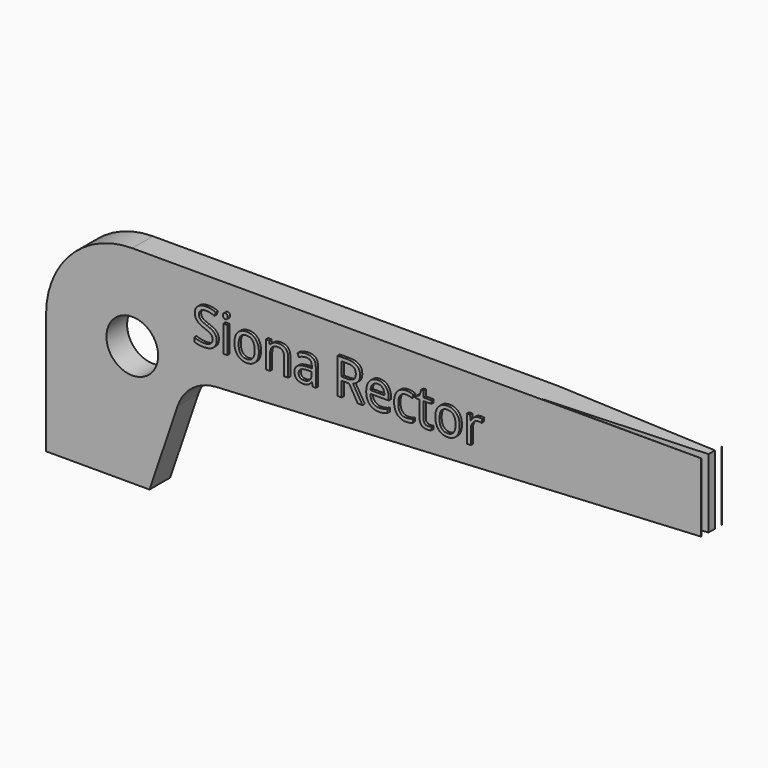
from build123d import *

# Parameters (mm, degrees)
F1_DEPTH     = 2.38125
F2_R         = 2.38125
F3_DEPTH     = 25.4
F6_DEPTH     = 25.4
F7_R         = 2.38125
F7_W         = 0.4099813808
F7_H         = 2.7055611352
F8_DEPTH     = 0.254
F9_TEXT_SIZE = 4.5757921827
F10_DEPTH    = 0.254


# Not quite as in the source:
# - Text() gives the source's letters only with a copy of the font that has no kerning and outlines rounded to 1/6400 em; it was checked with that copy


with BuildPart() as f1:
    # F0 (on Front) → F1 (new body)
    with BuildSketch(Plane.XZ):
        with BuildLine():
            Line((60.325, 19.05), (7.9375, 19.05))
            ThreePointArc((7.9375, 19.05), (2.3248399243, 16.7251600757), (0, 11.1125))
            Line((0, 11.1125), (0, 0))
            Line((0, 0), (9.525, 0))
            Line((9.525, 0), (12.1173647876, 7.6271664624))
            ThreePointArc((12.1173647876, 7.6271664624), (13.4786145605, 9.5135918491), (15.6631963617, 10.3130942181))
            Line((15.6631963617, 10.3130942181), (60.325, 12.7))
            Line((60.325, 12.7), (60.325, 19.05))
        make_face()
    extrude(amount=F1_DEPTH)

    # F2 (on face) → F3 (cut)
    with BuildSketch(Plane.XZ.offset(2.38125)):
        with Locations((7.9375, 11.1125)):
            Circle(F2_R)
    extrude(amount=-F3_DEPTH, mode=Mode.SUBTRACT)

    # F5 (on face) → F6 (cut)
    with BuildSketch(Plane.XY.offset(19.05)):
        Polygon((60.3245161474, 0), (45.24375, 0), (60.3431798518, -0.79375), align=None)
        Polygon((60.3431798518, -1.5423499767), (45.24375, -2.3360999767), (60.3328719735, -2.377419034), align=None)
    extrude(amount=-F6_DEPTH, mode=Mode.SUBTRACT)

    # F7 (on face) → F8 (cut)
    with BuildSketch(Plane.XZ.offset(2.38125)):
        with BuildLine():
            ThreePointArc((12.1173647876, 7.6271664624), (13.4786145605, 9.5135918491), (15.6631963617, 10.3130942181))
            Line((15.6631963617, 10.3130942181), (60.325, 12.7))
            Line((60.325, 12.7), (60.325, 19.05))
            Line((60.325, 19.05), (7.9375, 19.05))
            ThreePointArc((7.9375, 19.05), (2.3248399243, 16.7251600757), (0, 11.1125))
            Line((0, 11.1125), (0, 0))
            Line((0, 0), (9.525, 0))
            Line((9.525, 0), (12.1173647876, 7.6271664624))
        make_face()
        with Locations((7.9375, 11.1125)):
            Circle(F7_R, mode=Mode.SUBTRACT)
        with Locations((17.9440042047, 14.4853611236)):
            Rectangle(F7_W, F7_H, mode=Mode.SUBTRACT)
        with BuildLine():
            add(Edge.make_bspline(
                [(16.8487456605, 14.6950914831), (17.0620307718, 14.4628476951), (17.0620307718, 14.0931535021)],
                knots=[0, 0, 0, 1, 1, 1], degree=2))
            add(Edge.make_bspline(
                [(17.0620307718, 14.0931535021), (17.0620307718, 13.6168167533), (16.7164298969, 13.3498153916)],
                knots=[0, 0, 0, 1, 1, 1], degree=2))
            add(Edge.make_bspline(
                [(16.7164298969, 13.3498153916), (16.370829022, 13.08281403), (15.7783703792, 13.08281403)],
                knots=[0, 0, 0, 1, 1, 1], degree=2))
            add(Edge.make_bspline(
                [(15.7783703792, 13.08281403), (15.1369351554, 13.08281403), (14.790939308, 13.24870245)],
                knots=[0, 0, 0, 1, 1, 1], degree=2))
            Line((14.790939308, 13.24870245), (14.790939308, 13.6531542167))
            add(Edge.make_bspline(
                [(14.790939308, 13.6531542167), (15.0137037577, 13.5599407236), (15.2751755053, 13.5054345285)],
                knots=[0, 0, 0, 1, 1, 1], degree=2))
            add(Edge.make_bspline(
                [(15.2751755053, 13.5054345285), (15.536647253, 13.4509283333), (15.7933793315, 13.4509283333)],
                knots=[0, 0, 0, 1, 1, 1], degree=2))
            add(Edge.make_bspline(
                [(15.7933793315, 13.4509283333), (16.2128400506, 13.4509283333), (16.4253352171, 13.610102222)],
                knots=[0, 0, 0, 1, 1, 1], degree=2))
            add(Edge.make_bspline(
                [(16.4253352171, 13.610102222), (16.6378303836, 13.7692761107), (16.6378303836, 14.0536562592)],
                knots=[0, 0, 0, 1, 1, 1], degree=2))
            add(Edge.make_bspline(
                [(16.6378303836, 14.0536562592), (16.6378303836, 14.2408731903), (16.5623906498, 14.3605498362)],
                knots=[0, 0, 0, 1, 1, 1], degree=2))
            add(Edge.make_bspline(
                [(16.5623906498, 14.3605498362), (16.486950916, 14.480226482), (16.3103982404, 14.5817343961)],
                knots=[0, 0, 0, 1, 1, 1], degree=2))
            add(Edge.make_bspline(
                [(16.3103982404, 14.5817343961), (16.1338455649, 14.6832423102), (15.7736307101, 14.8112133771)],
                knots=[0, 0, 0, 1, 1, 1], degree=2))
            add(Edge.make_bspline(
                [(15.7736307101, 14.8112133771), (15.2704358362, 14.9913208045), (15.0543859178, 15.2381785723)],
                knots=[0, 0, 0, 1, 1, 1], degree=2))
            add(Edge.make_bspline(
                [(15.0543859178, 15.2381785723), (14.8383359994, 15.4850363401), (14.8383359994, 15.8823786031)],
                knots=[0, 0, 0, 1, 1, 1], degree=2))
            add(Edge.make_bspline(
                [(14.8383359994, 15.8823786031), (14.8383359994, 16.2994694876), (15.1515491352, 16.5463272554)],
                knots=[0, 0, 0, 1, 1, 1], degree=2))
            add(Edge.make_bspline(
                [(15.1515491352, 16.5463272554), (15.464762271, 16.7931850232), (15.9813862075, 16.7931850232)],
                knots=[0, 0, 0, 1, 1, 1], degree=2))
            add(Edge.make_bspline(
                [(15.9813862075, 16.7931850232), (16.5193386551, 16.7931850232), (16.9711871133, 16.595698809)],
                knots=[0, 0, 0, 1, 1, 1], degree=2))
            Line((16.9711871133, 16.595698809), (16.840056267, 16.2307442851))
            add(Edge.make_bspline(
                [(16.840056267, 16.2307442851), (16.392947478, 16.4179612162), (15.9711169243, 16.4179612162)],
                knots=[0, 0, 0, 1, 1, 1], degree=2))
            add(Edge.make_bspline(
                [(15.9711169243, 16.4179612162), (15.6377601947, 16.4179612162), (15.4501482912, 16.2749811971)],
                knots=[0, 0, 0, 1, 1, 1], degree=2))
            add(Edge.make_bspline(
                [(15.4501482912, 16.2749811971), (15.2625363876, 16.1320011779), (15.2625363876, 15.877638934)],
                knots=[0, 0, 0, 1, 1, 1], degree=2))
            add(Edge.make_bspline(
                [(15.2625363876, 15.877638934), (15.2625363876, 15.6904220029), (15.3316565626, 15.5703503846)],
                knots=[0, 0, 0, 1, 1, 1], degree=2))
            add(Edge.make_bspline(
                [(15.3316565626, 15.5703503846), (15.4007767376, 15.4502787664), (15.5650852679, 15.350350742)],
                knots=[0, 0, 0, 1, 1, 1], degree=2))
            add(Edge.make_bspline(
                [(15.5650852679, 15.350350742), (15.7293937981, 15.2504227175), (16.0674901969, 15.1295611544)],
                knots=[0, 0, 0, 1, 1, 1], degree=2))
            add(Edge.make_bspline(
                [(16.0674901969, 15.1295611544), (16.6354605491, 14.927335271), (16.8487456605, 14.6950914831)],
                knots=[0, 0, 0, 1, 1, 1], degree=2))
        make_face(mode=Mode.SUBTRACT)
        with BuildLine():
            add(Edge.make_bspline(
                [(21.018469588, 15.5099196031), (21.353011235, 15.131930989), (21.353011235, 14.4881259306)],
                knots=[0, 0, 0, 1, 1, 1], degree=2))
            add(Edge.make_bspline(
                [(21.353011235, 14.4881259306), (21.353011235, 13.8261521404), (21.0200494778, 13.4544830852)],
                knots=[0, 0, 0, 1, 1, 1], degree=2))
            add(Edge.make_bspline(
                [(21.0200494778, 13.4544830852), (20.6870877205, 13.08281403), (20.0993687469, 13.08281403)],
                knots=[0, 0, 0, 1, 1, 1], degree=2))
            add(Edge.make_bspline(
                [(20.0993687469, 13.08281403), (19.7359941127, 13.08281403), (19.4547737436, 13.2534421191)],
                knots=[0, 0, 0, 1, 1, 1], degree=2))
            add(Edge.make_bspline(
                [(19.4547737436, 13.2534421191), (19.1735533746, 13.4240702082), (19.0203040723, 13.7424179856)],
                knots=[0, 0, 0, 1, 1, 1], degree=2))
            add(Edge.make_bspline(
                [(19.0203040723, 13.7424179856), (18.86705477, 14.0607657629), (18.86705477, 14.4881259306)],
                knots=[0, 0, 0, 1, 1, 1], degree=2))
            add(Edge.make_bspline(
                [(18.86705477, 14.4881259306), (18.86705477, 15.1493097759), (19.1980416651, 15.5186089965)],
                knots=[0, 0, 0, 1, 1, 1], degree=2))
            add(Edge.make_bspline(
                [(19.1980416651, 15.5186089965), (19.5290285602, 15.8879082171), (20.1167475338, 15.8879082171)],
                knots=[0, 0, 0, 1, 1, 1], degree=2))
            add(Edge.make_bspline(
                [(20.1167475338, 15.8879082171), (20.6839279411, 15.8879082171), (21.018469588, 15.5099196031)],
                knots=[0, 0, 0, 1, 1, 1], degree=2))
        make_face(mode=Mode.SUBTRACT)
        with BuildLine():
            add(Edge.make_bspline(
                [(17.7733761156, 16.3650349108), (17.7042559406, 16.4329701685), (17.7042559406, 16.5712105184)],
                knots=[0, 0, 0, 1, 1, 1], degree=2))
            add(Edge.make_bspline(
                [(17.7042559406, 16.5712105184), (17.7042559406, 16.711820703), (17.7733761156, 16.7773861261)],
                knots=[0, 0, 0, 1, 1, 1], degree=2))
            add(Edge.make_bspline(
                [(17.7733761156, 16.7773861261), (17.8424962905, 16.8429515492), (17.9467690117, 16.8429515492)],
                knots=[0, 0, 0, 1, 1, 1], degree=2))
            add(Edge.make_bspline(
                [(17.9467690117, 16.8429515492), (18.0455121188, 16.8429515492), (18.1170021283, 16.7762012088)],
                knots=[0, 0, 0, 1, 1, 1], degree=2))
            add(Edge.make_bspline(
                [(18.1170021283, 16.7762012088), (18.1884921379, 16.7094508684), (18.1884921379, 16.5712105184)],
                knots=[0, 0, 0, 1, 1, 1], degree=2))
            add(Edge.make_bspline(
                [(18.1884921379, 16.5712105184), (18.1884921379, 16.4329701685), (18.1170021283, 16.3650349108)],
                knots=[0, 0, 0, 1, 1, 1], degree=2))
            add(Edge.make_bspline(
                [(18.1170021283, 16.3650349108), (18.0455121188, 16.2970996531), (17.9467690117, 16.2970996531)],
                knots=[0, 0, 0, 1, 1, 1], degree=2))
            add(Edge.make_bspline(
                [(17.9467690117, 16.2970996531), (17.8424962905, 16.2970996531), (17.7733761156, 16.3650349108)],
                knots=[0, 0, 0, 1, 1, 1], degree=2))
        make_face(mode=Mode.SUBTRACT)
        with BuildLine():
            Line((24.3334731804, 13.132580556), (23.9234917996, 13.132580556))
            Line((23.9234917996, 13.132580556), (23.9234917996, 14.8830983591))
            add(Edge.make_bspline(
                [(23.9234917996, 14.8830983591), (23.9234917996, 15.2132953093), (23.7730073043, 15.3764189222)],
                knots=[0, 0, 0, 1, 1, 1], degree=2))
            add(Edge.make_bspline(
                [(23.7730073043, 15.3764189222), (23.6225228091, 15.5395425352), (23.3010152523, 15.5395425352)],
                knots=[0, 0, 0, 1, 1, 1], degree=2))
            add(Edge.make_bspline(
                [(23.3010152523, 15.5395425352), (22.8768148641, 15.5395425352), (22.6793286499, 15.3100635543)],
                knots=[0, 0, 0, 1, 1, 1], degree=2))
            add(Edge.make_bspline(
                [(22.6793286499, 15.3100635543), (22.4818424356, 15.0805845733), (22.4818424356, 14.552111464)],
                knots=[0, 0, 0, 1, 1, 1], degree=2))
            Line((22.4818424356, 14.552111464), (22.4818424356, 13.132580556))
            Line((22.4818424356, 13.132580556), (22.0718610548, 13.132580556))
            Line((22.0718610548, 13.132580556), (22.0718610548, 15.8381416911))
            Line((22.0718610548, 15.8381416911), (22.4052177845, 15.8381416911))
            Line((22.4052177845, 15.8381416911), (22.4715731525, 15.4676575532))
            Line((22.4715731525, 15.4676575532), (22.4913217739, 15.4676575532))
            add(Edge.make_bspline(
                [(22.4913217739, 15.4676575532), (22.617712951, 15.667513602), (22.8448220974, 15.7777109096)],
                knots=[0, 0, 0, 1, 1, 1], degree=2))
            add(Edge.make_bspline(
                [(22.8448220974, 15.7777109096), (23.0719312438, 15.8879082171), (23.3507817783, 15.8879082171)],
                knots=[0, 0, 0, 1, 1, 1], degree=2))
            add(Edge.make_bspline(
                [(23.3507817783, 15.8879082171), (23.8397576448, 15.8879082171), (24.0866154126, 15.6521096773)],
                knots=[0, 0, 0, 1, 1, 1], degree=2))
            add(Edge.make_bspline(
                [(24.0866154126, 15.6521096773), (24.3334731804, 15.4163111375), (24.3334731804, 14.8973173665)],
                knots=[0, 0, 0, 1, 1, 1], degree=2))
            Line((24.3334731804, 14.8973173665), (24.3334731804, 13.132580556))
        make_face(mode=Mode.SUBTRACT)
        with BuildLine():
            Line((27.1425170918, 13.132580556), (26.8383883219, 13.132580556))
            Line((26.8383883219, 13.132580556), (26.7570240016, 13.5180736462))
            Line((26.7570240016, 13.5180736462), (26.7372753802, 13.5180736462))
            add(Edge.make_bspline(
                [(26.7372753802, 13.5180736462), (26.5350494968, 13.2637114022), (26.3340085307, 13.1732627161)],
                knots=[0, 0, 0, 1, 1, 1], degree=2))
            add(Edge.make_bspline(
                [(26.3340085307, 13.1732627161), (26.1329675646, 13.08281403), (25.8312086292, 13.08281403)],
                knots=[0, 0, 0, 1, 1, 1], degree=2))
            add(Edge.make_bspline(
                [(25.8312086292, 13.08281403), (25.429126697, 13.08281403), (25.2008326333, 13.2905695274)],
                knots=[0, 0, 0, 1, 1, 1], degree=2))
            add(Edge.make_bspline(
                [(25.2008326333, 13.2905695274), (24.9725385697, 13.4983250248), (24.9725385697, 13.8806583355)],
                knots=[0, 0, 0, 1, 1, 1], degree=2))
            add(Edge.make_bspline(
                [(24.9725385697, 13.8806583355), (24.9725385697, 14.6998311522), (26.2830570874, 14.7393283951)],
                knots=[0, 0, 0, 1, 1, 1], degree=2))
            Line((26.2830570874, 14.7393283951), (26.7420150493, 14.7543373474))
            Line((26.7420150493, 14.7543373474), (26.7420150493, 14.9225956019))
            add(Edge.make_bspline(
                [(26.7420150493, 14.9225956019), (26.7420150493, 15.2409433793), (26.6053545891, 15.3926127918)],
                knots=[0, 0, 0, 1, 1, 1], degree=2))
            add(Edge.make_bspline(
                [(26.6053545891, 15.3926127918), (26.4686941288, 15.5442822043), (26.1669351934, 15.5442822043)],
                knots=[0, 0, 0, 1, 1, 1], degree=2))
            add(Edge.make_bspline(
                [(26.1669351934, 15.5442822043), (25.8288387946, 15.5442822043), (25.4022685719, 15.3373166518)],
                knots=[0, 0, 0, 1, 1, 1], degree=2))
            Line((25.4022685719, 15.3373166518), (25.2758773948, 15.65092476))
            add(Edge.make_bspline(
                [(25.2758773948, 15.65092476), (25.4757334436, 15.7591472054), (25.713901818, 15.8207629043)],
                knots=[0, 0, 0, 1, 1, 1], degree=2))
            add(Edge.make_bspline(
                [(25.713901818, 15.8207629043), (25.9520701923, 15.8823786031), (26.1922134289, 15.8823786031)],
                knots=[0, 0, 0, 1, 1, 1], degree=2))
            add(Edge.make_bspline(
                [(26.1922134289, 15.8823786031), (26.6756596813, 15.8823786031), (26.9090883866, 15.6679085745)],
                knots=[0, 0, 0, 1, 1, 1], degree=2))
            add(Edge.make_bspline(
                [(26.9090883866, 15.6679085745), (27.1425170918, 15.4534385458), (27.1425170918, 14.9794716316)],
                knots=[0, 0, 0, 1, 1, 1], degree=2))
            Line((27.1425170918, 14.9794716316), (27.1425170918, 13.132580556))
        make_face(mode=Mode.SUBTRACT)
        with BuildLine():
            add(Edge.make_bspline(
                [(34.0355759139, 13.1238911625), (33.8420394239, 13.08281403), (33.5679285585, 13.08281403)],
                knots=[0, 0, 0, 1, 1, 1], degree=2))
            add(Edge.make_bspline(
                [(33.5679285585, 13.08281403), (32.9683604121, 13.08281403), (32.6211796474, 13.4485584988)],
                knots=[0, 0, 0, 1, 1, 1], degree=2))
            add(Edge.make_bspline(
                [(32.6211796474, 13.4485584988), (32.2739988828, 13.8143029676), (32.2739988828, 14.4628476951)],
                knots=[0, 0, 0, 1, 1, 1], degree=2))
            add(Edge.make_bspline(
                [(32.2739988828, 14.4628476951), (32.2739988828, 15.1177119816), (32.5962963844, 15.5028100994)],
                knots=[0, 0, 0, 1, 1, 1], degree=2))
            add(Edge.make_bspline(
                [(32.5962963844, 15.5028100994), (32.9185938861, 15.8879082171), (33.4620759477, 15.8879082171)],
                knots=[0, 0, 0, 1, 1, 1], degree=2))
            add(Edge.make_bspline(
                [(33.4620759477, 15.8879082171), (33.9700104907, 15.8879082171), (34.2662398121, 15.5533665702)],
                knots=[0, 0, 0, 1, 1, 1], degree=2))
            add(Edge.make_bspline(
                [(34.2662398121, 15.5533665702), (34.5624691335, 15.2188249233), (34.5624691335, 14.6706031925)],
                knots=[0, 0, 0, 1, 1, 1], degree=2))
            Line((34.5624691335, 14.6706031925), (34.5624691335, 14.4115012794))
            Line((34.5624691335, 14.4115012794), (32.6989892158, 14.4115012794))
            add(Edge.make_bspline(
                [(32.6989892158, 14.4115012794), (32.7116283335, 13.9351645307), (32.9399223972, 13.6883067629)],
                knots=[0, 0, 0, 1, 1, 1], degree=2))
            add(Edge.make_bspline(
                [(32.9399223972, 13.6883067629), (33.1682164609, 13.4414489951), (33.5829375108, 13.4414489951)],
                knots=[0, 0, 0, 1, 1, 1], degree=2))
            add(Edge.make_bspline(
                [(33.5829375108, 13.4414489951), (34.0197770167, 13.4414489951), (34.4463472395, 13.623926257)],
                knots=[0, 0, 0, 1, 1, 1], degree=2))
            Line((34.4463472395, 13.623926257), (34.4463472395, 13.2581817882))
            add(Edge.make_bspline(
                [(34.4463472395, 13.2581817882), (34.2291124038, 13.1649682951), (34.0355759139, 13.1238911625)],
                knots=[0, 0, 0, 1, 1, 1], degree=2))
        make_face(mode=Mode.SUBTRACT)
        with BuildLine():
            Line((30.5345403077, 14.6334757842), (29.7809329141, 14.6334757842))
            Line((29.7809329141, 14.6334757842), (29.7809329141, 13.132580556))
            Line((29.7809329141, 13.132580556), (29.3614721951, 13.132580556))
            Line((29.3614721951, 13.132580556), (29.3614721951, 16.7418386075))
            Line((29.3614721951, 16.7418386075), (30.3512731009, 16.7418386075))
            add(Edge.make_bspline(
                [(30.3512731009, 16.7418386075), (31.0156167256, 16.7418386075), (31.3327795857, 16.4874763636)],
                knots=[0, 0, 0, 1, 1, 1], degree=2))
            add(Edge.make_bspline(
                [(31.3327795857, 16.4874763636), (31.6499424458, 16.2331141196), (31.6499424458, 15.7220197972)],
                knots=[0, 0, 0, 1, 1, 1], degree=2))
            add(Edge.make_bspline(
                [(31.6499424458, 15.7220197972), (31.6499424458, 15.0063297567), (30.9239831222, 14.7543373474)],
                knots=[0, 0, 0, 1, 1, 1], degree=2))
            Line((30.9239831222, 14.7543373474), (31.9043046897, 13.132580556))
            Line((31.9043046897, 13.132580556), (31.4082193195, 13.132580556))
            Line((31.4082193195, 13.132580556), (30.5345403077, 14.6334757842))
        make_face(mode=Mode.SUBTRACT)
        with BuildLine():
            add(Edge.make_bspline(
                [(37.0263071424, 13.2242141594), (36.7553560564, 13.08281403), (36.3430048411, 13.08281403)],
                knots=[0, 0, 0, 1, 1, 1], degree=2))
            add(Edge.make_bspline(
                [(36.3430048411, 13.08281403), (35.7552858675, 13.08281403), (35.4329883659, 13.4446087745)],
                knots=[0, 0, 0, 1, 1, 1], degree=2))
            add(Edge.make_bspline(
                [(35.4329883659, 13.4446087745), (35.1106908642, 13.806403519), (35.1106908642, 14.4683773091)],
                knots=[0, 0, 0, 1, 1, 1], degree=2))
            add(Edge.make_bspline(
                [(35.1106908642, 14.4683773091), (35.1106908642, 15.1469399413), (35.4381230074, 15.5174240792)],
                knots=[0, 0, 0, 1, 1, 1], degree=2))
            add(Edge.make_bspline(
                [(35.4381230074, 15.5174240792), (35.7655551506, 15.8879082171), (36.3698629662, 15.8879082171)],
                knots=[0, 0, 0, 1, 1, 1], degree=2))
            add(Edge.make_bspline(
                [(36.3698629662, 15.8879082171), (36.5649793459, 15.8879082171), (36.7600957256, 15.8456461673)],
                knots=[0, 0, 0, 1, 1, 1], degree=2))
            add(Edge.make_bspline(
                [(36.7600957256, 15.8456461673), (36.9552121053, 15.8033841174), (37.0658043852, 15.7465080877)],
                knots=[0, 0, 0, 1, 1, 1], degree=2))
            Line((37.0658043852, 15.7465080877), (36.940203153, 15.3989323507))
            add(Edge.make_bspline(
                [(36.940203153, 15.3989323507), (36.8043326376, 15.4534385458), (36.6439738316, 15.4889860644)],
                knots=[0, 0, 0, 1, 1, 1], degree=2))
            add(Edge.make_bspline(
                [(36.6439738316, 15.4889860644), (36.4836150256, 15.5245335829), (36.360383628, 15.5245335829)],
                knots=[0, 0, 0, 1, 1, 1], degree=2))
            add(Edge.make_bspline(
                [(36.360383628, 15.5245335829), (35.5356811973, 15.5245335829), (35.5356811973, 14.4731169783)],
                knots=[0, 0, 0, 1, 1, 1], degree=2))
            add(Edge.make_bspline(
                [(35.5356811973, 14.4731169783), (35.5356811973, 13.9746617735), (35.7367221634, 13.7080553843)],
                knots=[0, 0, 0, 1, 1, 1], degree=2))
            add(Edge.make_bspline(
                [(35.7367221634, 13.7080553843), (35.9377631295, 13.4414489951), (36.332735558, 13.4414489951)],
                knots=[0, 0, 0, 1, 1, 1], degree=2))
            add(Edge.make_bspline(
                [(36.332735558, 13.4414489951), (36.6708319568, 13.4414489951), (37.0263071424, 13.5867988487)],
                knots=[0, 0, 0, 1, 1, 1], degree=2))
            Line((37.0263071424, 13.5867988487), (37.0263071424, 13.2242141594))
        make_face(mode=Mode.SUBTRACT)
        with BuildLine():
            add(Edge.make_bspline(
                [(38.2238635456, 13.5524362475), (38.3399854396, 13.4217003736), (38.5422113229, 13.4217003736)],
                knots=[0, 0, 0, 1, 1, 1], degree=2))
            add(Edge.make_bspline(
                [(38.5422113229, 13.4217003736), (38.6512237132, 13.4217003736), (38.7523366549, 13.4374992708)],
                knots=[0, 0, 0, 1, 1, 1], degree=2))
            add(Edge.make_bspline(
                [(38.7523366549, 13.4374992708), (38.8534495966, 13.4532981679), (38.9126954609, 13.4706769548)],
                knots=[0, 0, 0, 1, 1, 1], degree=2))
            Line((38.9126954609, 13.4706769548), (38.9126954609, 13.1570688465))
            add(Edge.make_bspline(
                [(38.9126954609, 13.1570688465), (38.8463400929, 13.1254710523), (38.7167891363, 13.1041425411)],
                knots=[0, 0, 0, 1, 1, 1], degree=2))
            add(Edge.make_bspline(
                [(38.7167891363, 13.1041425411), (38.5872381798, 13.08281403), (38.4829654587, 13.08281403)],
                knots=[0, 0, 0, 1, 1, 1], degree=2))
            add(Edge.make_bspline(
                [(38.4829654587, 13.08281403), (37.6985502157, 13.08281403), (37.6985502157, 13.9098862952)],
                knots=[0, 0, 0, 1, 1, 1], degree=2))
            Line((37.6985502157, 13.9098862952), (37.6985502157, 15.5197939138))
            Line((37.6985502157, 15.5197939138), (37.3106872909, 15.5197939138))
            Line((37.3106872909, 15.5197939138), (37.3106872909, 15.717280128))
            Line((37.3106872909, 15.717280128), (37.6985502157, 15.8879082171))
            Line((37.6985502157, 15.8879082171), (37.8707581945, 16.4653579076))
            Line((37.8707581945, 16.4653579076), (38.1077416516, 16.4653579076))
            Line((38.1077416516, 16.4653579076), (38.1077416516, 15.8381416911))
            Line((38.1077416516, 15.8381416911), (38.8929468394, 15.8381416911))
            Line((38.8929468394, 15.8381416911), (38.8929468394, 15.5197939138))
            Line((38.8929468394, 15.5197939138), (38.1077416516, 15.5197939138))
            Line((38.1077416516, 15.5197939138), (38.1077416516, 13.9272650821))
            add(Edge.make_bspline(
                [(38.1077416516, 13.9272650821), (38.1077416516, 13.6831721213), (38.2238635456, 13.5524362475)],
                knots=[0, 0, 0, 1, 1, 1], degree=2))
        make_face(mode=Mode.SUBTRACT)
        with BuildLine():
            add(Edge.make_bspline(
                [(41.4535530934, 15.5099196031), (41.7880947403, 15.131930989), (41.7880947403, 14.4881259306)],
                knots=[0, 0, 0, 1, 1, 1], degree=2))
            add(Edge.make_bspline(
                [(41.7880947403, 14.4881259306), (41.7880947403, 13.8261521404), (41.4551329831, 13.4544830852)],
                knots=[0, 0, 0, 1, 1, 1], degree=2))
            add(Edge.make_bspline(
                [(41.4551329831, 13.4544830852), (41.1221712259, 13.08281403), (40.5344522523, 13.08281403)],
                knots=[0, 0, 0, 1, 1, 1], degree=2))
            add(Edge.make_bspline(
                [(40.5344522523, 13.08281403), (40.171077618, 13.08281403), (39.889857249, 13.2534421191)],
                knots=[0, 0, 0, 1, 1, 1], degree=2))
            add(Edge.make_bspline(
                [(39.889857249, 13.2534421191), (39.6086368799, 13.4240702082), (39.4553875776, 13.7424179856)],
                knots=[0, 0, 0, 1, 1, 1], degree=2))
            add(Edge.make_bspline(
                [(39.4553875776, 13.7424179856), (39.3021382754, 14.0607657629), (39.3021382754, 14.4881259306)],
                knots=[0, 0, 0, 1, 1, 1], degree=2))
            add(Edge.make_bspline(
                [(39.3021382754, 14.4881259306), (39.3021382754, 15.1493097759), (39.6331251704, 15.5186089965)],
                knots=[0, 0, 0, 1, 1, 1], degree=2))
            add(Edge.make_bspline(
                [(39.6331251704, 15.5186089965), (39.9641120655, 15.8879082171), (40.5518310391, 15.8879082171)],
                knots=[0, 0, 0, 1, 1, 1], degree=2))
            add(Edge.make_bspline(
                [(40.5518310391, 15.8879082171), (41.1190114464, 15.8879082171), (41.4535530934, 15.5099196031)],
                knots=[0, 0, 0, 1, 1, 1], degree=2))
        make_face(mode=Mode.SUBTRACT)
        with BuildLine():
            add(Edge.make_bspline(
                [(43.2747709611, 15.7445332256), (43.4872661277, 15.8879082171), (43.7416283716, 15.8879082171)],
                knots=[0, 0, 0, 1, 1, 1], degree=2))
            add(Edge.make_bspline(
                [(43.7416283716, 15.8879082171), (43.921735799, 15.8879082171), (44.0647158181, 15.8578903126)],
                knots=[0, 0, 0, 1, 1, 1], degree=2))
            Line((44.0647158181, 15.8578903126), (44.0078397884, 15.4779268364))
            add(Edge.make_bspline(
                [(44.0078397884, 15.4779268364), (43.8403714787, 15.5150542446), (43.711610467, 15.5150542446)],
                knots=[0, 0, 0, 1, 1, 1], degree=2))
            add(Edge.make_bspline(
                [(43.711610467, 15.5150542446), (43.3829934065, 15.5150542446), (43.1499596737, 15.2484478554)],
                knots=[0, 0, 0, 1, 1, 1], degree=2))
            add(Edge.make_bspline(
                [(43.1499596737, 15.2484478554), (42.9169259409, 14.9818414662), (42.9169259409, 14.5844992031)],
                knots=[0, 0, 0, 1, 1, 1], degree=2))
            Line((42.9169259409, 14.5844992031), (42.9169259409, 13.132580556))
            Line((42.9169259409, 13.132580556), (42.5069445601, 13.132580556))
            Line((42.5069445601, 13.132580556), (42.5069445601, 15.8381416911))
            Line((42.5069445601, 15.8381416911), (42.8450409589, 15.8381416911))
            Line((42.8450409589, 15.8381416911), (42.8924376504, 15.3373166518))
            Line((42.8924376504, 15.3373166518), (42.9121862718, 15.3373166518))
            add(Edge.make_bspline(
                [(42.9121862718, 15.3373166518), (43.0622757946, 15.601158234), (43.2747709611, 15.7445332256)],
                knots=[0, 0, 0, 1, 1, 1], degree=2))
        make_face(mode=Mode.SUBTRACT)
    extrude(amount=F8_DEPTH, mode=Mode.SUBTRACT)

    # F9 (on face) → F10 (join)
    with BuildSketch(Plane.XZ.offset(2.38125)):
        with Locations((13.6199574918, 13.386964798)):
            Text('Siona Rector', F9_TEXT_SIZE, font='Open Sans', text_align=(TextAlign.LEFT, TextAlign.BOTTOM))
    extrude(amount=F10_DEPTH)


solid = f1.part
